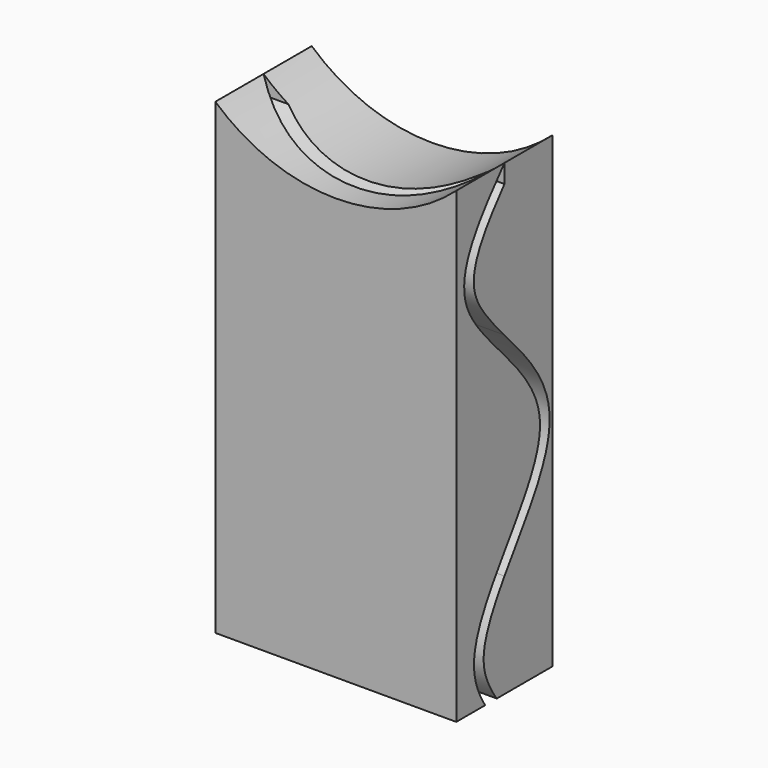
from build123d import *

# Parameters (mm, degrees)
F0_W     = 50.8
F0_H     = 25.4
F1_DEPTH = 127
F3_DEPTH = 99.568
F5_DEPTH = 87.63


# Not quite as in the source:
# - the dataset's text gives a spline's control points without its knots; the knots are read off the source's solid


with BuildPart() as f1:
    # F0 (on Top) → F1 (new body)
    with BuildSketch(Plane.XY):
        with Locations((25.4, 12.7)):
            Rectangle(F0_W, F0_H)
    extrude(amount=F1_DEPTH)

    # F2 (on face) → F3 (cut)
    with BuildSketch(Plane(origin=(0, 25.4, 0), x_dir=(-1, 0, 0), z_dir=(0, 1, 0))):
        with BuildLine():
            Line((-50.8, 127), (-50.8, 98.6019366858))
            ThreePointArc((-50.8, 98.6019366858), (-25.4, 88.9), (0, 98.6019366858))
            Line((0, 98.6019366858), (0, 127))
            Line((0, 127), (-50.8, 127))
        make_face()
    extrude(amount=-F3_DEPTH, mode=Mode.SUBTRACT)

    # F4 (on face) → F5 (cut)
    with BuildSketch(Plane.YZ.offset(50.8)):
        with BuildLine():
            Line((12.7, 94.6786641578), (12.7, 98.6019366858))
            add(Edge.make_bspline(
                [(12.7, 98.6019366858), (6.3941442473, 91.2167877182), (-3.4982772544, 79.6312061087), (8.4931261842, 67.5038075354), (12.7, 62.8944715835)],
                knots=[0, 0, 0, 0, 0.1751950427, 0.2748402875, 0.2748402875, 0.2748402875, 0.2748402875], degree=3))
            Line((12.7, 62.8944715835), (12.7, 66.6492583242))
            add(Edge.make_bspline(
                [(12.7, 94.6786641578), (12.2397414191, 94.1312347125), (10.711066967, 92.2921912432), (8.3238323958, 89.2117149421), (6.4284756304, 86.1437293907), (5.3847824977, 83.8025497315), (4.8589372168, 82.1157305832), (4.601213696, 80.50130944), (4.6129315615, 79.2012257855), (4.7663046406, 78.1651542281), (4.958272825, 77.3824904778), (5.2342351085, 76.5878188669), (5.6093004495, 75.7466319011), (6.0788246889, 74.8690486526), (6.8249665125, 73.6550882454), (8.4223872761, 71.4327598786), (10.5741233601, 68.9676707912), (12.2790443941, 67.1071580514), (12.7, 66.6492583242)],
                knots=[0.0180956937, 0.0180956937, 0.0180956937, 0.0180956937, 0.03125, 0.0625, 0.09375, 0.109375, 0.125, 0.140625, 0.15625, 0.1640625, 0.171875, 0.1796875, 0.1875, 0.1953125, 0.203125, 0.21875, 0.25, 0.2600729194, 0.2600729194, 0.2600729194, 0.2600729194], degree=3))
        make_face()
        with BuildLine():
            Line((12.7, 66.6492583242), (12.7, 62.8944715835))
            add(Edge.make_bspline(
                [(12.7, 62.8944715835), (17.394992931, 57.7503192609), (26.7747840396, 46.5255516353), (17.336611886, 33.3155088327), (12.7, 26.480417506)],
                knots=[0.2748402875, 0.2748402875, 0.2748402875, 0.2748402875, 0.3860472645, 0.5056265986, 0.5056265986, 0.5056265986, 0.5056265986], degree=3))
            Line((12.7, 26.480417506), (12.7, 21.9024276787))
            add(Edge.make_bspline(
                [(12.7, 66.6492583242), (13.5850076531, 65.6865801766), (15.8346538576, 63.2554060867), (18.7091009815, 59.9372449221), (21.0307282182, 56.7066450653), (22.537625948, 54.169749137), (23.5274792553, 51.9392454559), (24.1079193054, 50.0751355096), (24.422175727, 48.6371958766), (24.6007289351, 47.1621716676), (24.6254251639, 45.654756511), (24.4995897033, 44.165436997), (24.1568489788, 42.2010675274), (23.4391648092, 39.7926811719), (22.2245527821, 36.9645450433), (20.743720073, 34.1807423385), (18.516613048, 30.5128624802), (15.714409274, 26.3989259536), (13.5791806325, 23.2559774163), (12.7, 21.9024276787)],
                knots=[0.2600729194, 0.2600729194, 0.2600729194, 0.2600729194, 0.28125, 0.3125, 0.328125, 0.34375, 0.359375, 0.3671875, 0.375, 0.3828125, 0.390625, 0.3984375, 0.40625, 0.421875, 0.4375, 0.453125, 0.46875, 0.5, 0.5242712372, 0.5242712372, 0.5242712372, 0.5242712372], degree=3))
        make_face()
        with BuildLine():
            Line((12.7, 21.9024276787), (12.7, 26.480417506))
            add(Edge.make_bspline(
                [(12.7, 26.480417506), (8.4252401598, 20.1787527071), (2.448928877, 10.9126897812), (5.9531043263, 2.5858334837), (7.6043491835, 0)],
                knots=[0.5056265986, 0.5056265986, 0.5056265986, 0.5056265986, 0.6158736815, 0.6679445301, 0.6679445301, 0.6679445301, 0.6679445301], degree=3))
            Line((7.6043491835, 0), (10.6747954064, 0))
            add(Edge.make_bspline(
                [(12.7, 21.9024276787), (12.4472072391, 21.5132385148), (11.6429519427, 20.258141903), (10.3810320273, 18.1685346385), (9.0699160822, 15.6827660293), (8.0601171051, 13.2992644725), (7.4060517856, 11.0489840471), (7.2075067484, 9.4824526121), (7.200844971, 8.4852964821), (7.2301369182, 7.8340119196), (7.3719787133, 6.6901029654), (7.8276275834, 5.0218449334), (8.762341912, 2.9532745811), (9.7856800938, 1.2670621413), (10.4747820792, 0.2779354298), (10.6747954064, 0)],
                knots=[0.5242712372, 0.5242712372, 0.5242712372, 0.5242712372, 0.53125, 0.546875, 0.5625, 0.578125, 0.59375, 0.609375, 0.61328125, 0.6171875, 0.625, 0.640625, 0.65625, 0.671875, 0.6779663373, 0.6779663373, 0.6779663373, 0.6779663373], degree=3))
        make_face()
    extrude(amount=-F5_DEPTH, mode=Mode.SUBTRACT)


solid = f1.part
